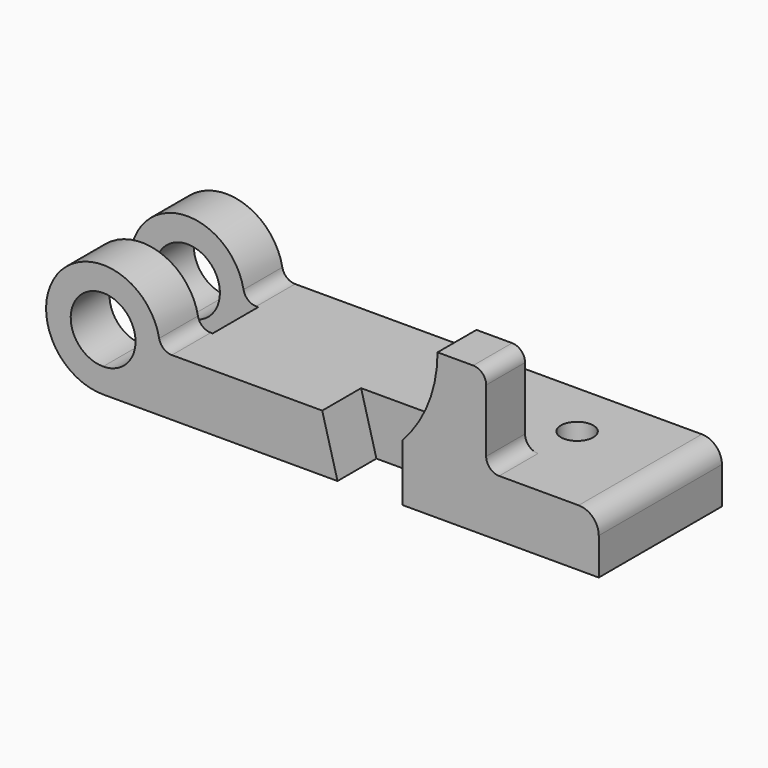
from build123d import *

# Parameters (mm, degrees)
F1_DEPTH = 30.1625
F0_W     = 19.05
F0_H     = 34.798
F2_DEPTH = 30.1625
F3_DEPTH = 11.1125
F4_R     = 6.35
F5_DEPTH = 22.353
F7_DEPTH = 19.05
F8_W     = 114.3
F8_H     = 22.3266
F9_DEPTH = 88.9
F10_R    = 5.08
F11_R    = 7.874


with BuildPart() as f1:
    # F0 (on Front) → F1 (new body, symmetric)
    with BuildSketch(Plane.XZ):
        with BuildLine():
            ThreePointArc((-97.1042, -1.524), (-106.084456, 20.156256), (-84.4042, 11.176))
            Line((-84.4042, 11.176), (-74.7522, 11.176))
            ThreePointArc((-74.7522, 11.176), (-112.909451, 26.981251), (-97.1042, -11.176))
            Line((-97.1042, -11.176), (-97.1042, -1.524))
        make_face()
        with BuildLine():
            Line((-74.7522, 11.176), (-84.4042, 11.176))
            ThreePointArc((-84.4042, 11.176), (-88.123944, 2.195744), (-97.1042, -1.524))
            Line((-97.1042, -1.524), (-97.1042, -11.176))
            ThreePointArc((-97.1042, -11.176), (-81.298949, -4.629251), (-74.7522, 11.176))
        make_face()
        with BuildLine():
            Line((-11.2522, 11.176), (-74.7522, 11.176))
            ThreePointArc((-74.7522, 11.176), (-81.298949, -4.629251), (-97.1042, -11.176))
            Line((-97.1042, -11.176), (-5.2578, -11.176))
            Line((-5.2578, -11.176), (-11.2522, 11.176))
        make_face()
        Polygon((20.1422, 11.176), (-11.2522, 11.176), (-5.2578, -11.176), (20.1422, -11.176), (20.1422, 11.173673), align=None)
        with BuildLine():
            Line((20.1422, 11.173673), (20.1422, -11.176))
            Line((20.1422, -11.176), (97.1042, -11.176))
            Line((97.1042, -11.176), (97.1042, 11.176))
            Line((97.1042, 11.176), (52.9844, 11.176))
            Line((52.9844, 11.176), (33.9344, 11.176))
            Line((33.9344, 11.176), (20.144388, 11.176))
            ThreePointArc((20.144388, 11.176), (20.143294, 11.174837), (20.1422, 11.173673))
        make_face()
    extrude(amount=F1_DEPTH, both=True)

    # F0 (on Front) → F2 (join)
    with BuildSketch(Plane.XZ):
        with Locations((43.4594, 28.575)):
            Rectangle(F0_W, F0_H)
        with BuildLine():
            ThreePointArc((33.9344, 45.974), (30.361232, 27.258597), (20.144388, 11.176))
            Line((20.144388, 11.176), (33.9344, 11.176))
            Line((33.9344, 11.176), (33.9344, 45.974))
        make_face()
    extrude(amount=F2_DEPTH)

    # F0 (on Front) → F3 (cut)
    with BuildSketch(Plane.XZ):
        with Locations((43.4594, 28.575)):
            Rectangle(F0_W, F0_H)
        with BuildLine():
            ThreePointArc((33.9344, 45.974), (30.361232, 27.258597), (20.144388, 11.176))
            Line((20.144388, 11.176), (33.9344, 11.176))
            Line((33.9344, 11.176), (33.9344, 45.974))
        make_face()
    extrude(amount=F3_DEPTH, mode=Mode.SUBTRACT)

    # F4 (on face) → F5 (cut, through all)
    with BuildSketch(Plane.XY.offset(11.176)):
        with Locations((58.2422, 7.8105)):
            Circle(F4_R)
    extrude(amount=-F5_DEPTH, mode=Mode.SUBTRACT)

    # F6 (on face) → F7 (cut)
    with BuildSketch(Plane.XZ.offset(30.1625)):
        Polygon((20.1422, -11.176), (20.1422, 11.173673), (20.1422, 11.176), (-11.2522, 11.176), (-5.2578, -11.176), align=None)
    extrude(amount=-F7_DEPTH, mode=Mode.SUBTRACT)

    # F8 (on Top) → F9 (cut, symmetric)
    with BuildSketch(Plane.XY):
        with Locations((-126.525862, 0)):
            Rectangle(F8_W, F8_H)
    extrude(amount=F9_DEPTH, both=True, mode=Mode.SUBTRACT)

    # F10
    f10_edges = [f1.edges().sort_by_distance(p)[0] for p in [
        (-74.7522, 20.6629, 11.176),
        (-74.7522, -20.6629, 11.176),
        (52.9844, -20.6375, 11.176),
        (52.9844, -20.6375, 45.974),
    ]]
    fillet(f10_edges, radius=F10_R)

    # F11
    f11_edges = [f1.edges().sort_by_distance(p)[0] for p in [
        (97.1042, 0, 11.176),
    ]]
    fillet(f11_edges, radius=F11_R)


solid = f1.part
